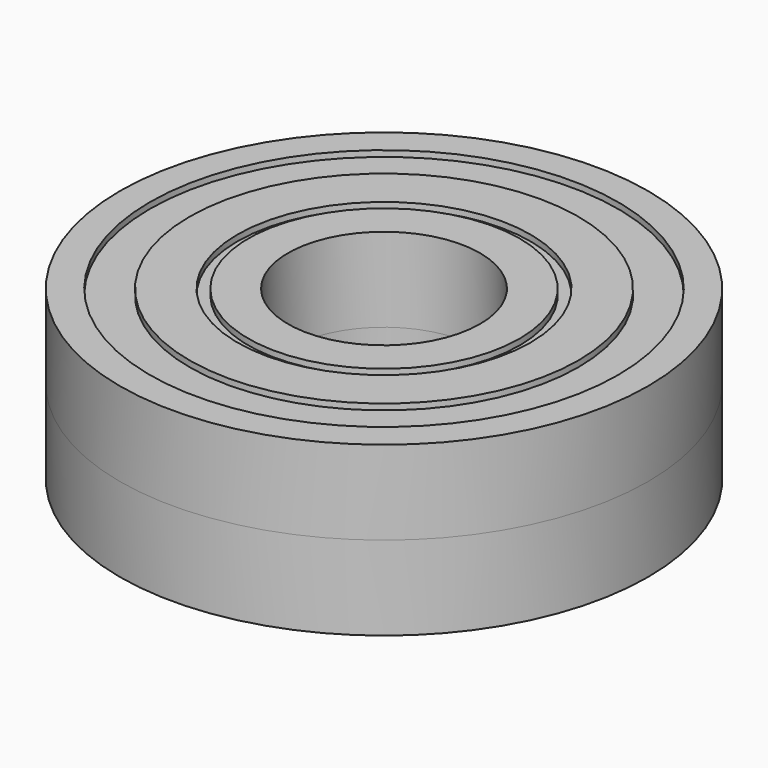
from build123d import *

# Parameters (mm, degrees)
F0_R     = 11
F0_R_2   = 9.75
F0_R_3   = 8.1
F0_R_4   = 6.1
F0_R_5   = 5.65
F0_R_6   = 4
F1_DEPTH = 3.5
F2_DEPTH = 0.25


with BuildPart() as f1:
    # F0 (on Top) → F1 (new body)
    with BuildSketch(Plane.XY):
        Circle(F0_R)
        Circle(F0_R_2, mode=Mode.SUBTRACT)
        Circle(F0_R_2)
        Circle(F0_R_3, mode=Mode.SUBTRACT)
        Circle(F0_R_3)
        Circle(F0_R_4, mode=Mode.SUBTRACT)
        Circle(F0_R_4)
        Circle(F0_R_5, mode=Mode.SUBTRACT)
        Circle(F0_R_5)
        Circle(F0_R_6, mode=Mode.SUBTRACT)
    extrude(amount=F1_DEPTH)

    # F0 (on Top) → F2 (cut)
    with BuildSketch(Plane.XY):
        Circle(F0_R_2)
        Circle(F0_R_3, mode=Mode.SUBTRACT)
        Circle(F0_R_4)
        Circle(F0_R_5, mode=Mode.SUBTRACT)
    extrude(amount=F2_DEPTH, mode=Mode.SUBTRACT)

    # F3: F1 across face


with BuildPart() as f1_1:
    add(f1.part)
    add(f1.part.mirror(Plane.XY.offset(3.5)))


solid = f1_1.part
